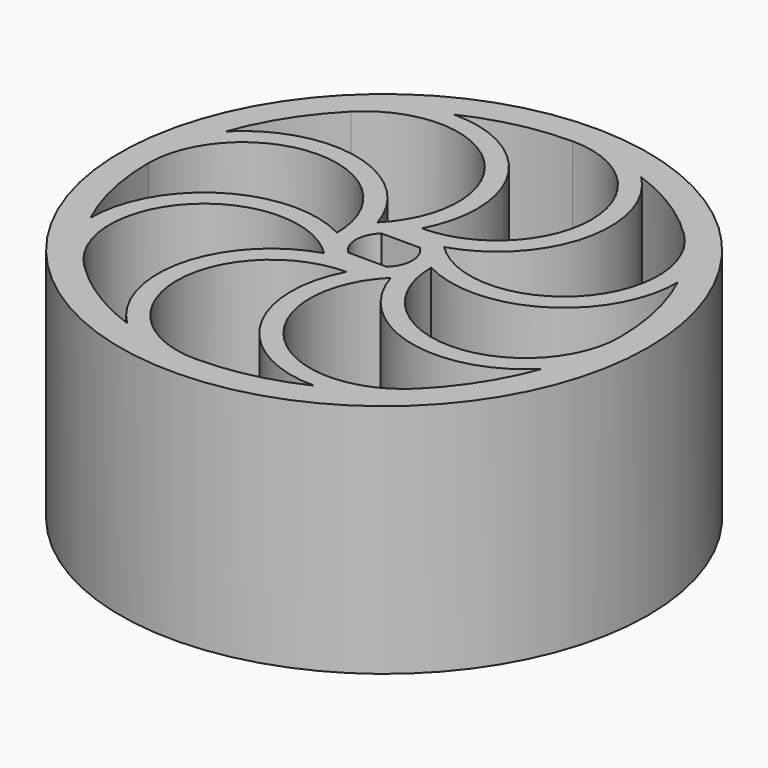
from build123d import *

# Parameters (mm, degrees)
F0_R     = 28
F1_DEPTH = 25
F2_W     = 4.0792156109
F2_H     = 4.4
F3_DEPTH = 30
F4_R     = 5
F4_R_2   = 3.5
F5_DEPTH = 1


# Not quite as in the source:
# - ends of sketch curves that miss each other by under 0.0002 mm in the source are joined


with BuildPart() as f1:
    # F0 (on Top) → F1 (new body)
    with BuildSketch(Plane.XY):
        Circle(F0_R)
        with BuildLine():
            ThreePointArc((22.6064085074, 10.6747503202), (24.3942638, 5.4699080119), (25, 0))
            ThreePointArc((25, 0), (24.6306042082, -4.2817445441), (23.5333330927, -8.4369564149))
            ThreePointArc((23.5333330927, -8.4369564149), (21.1171584026, -13.3815403074), (17.6776695297, -17.6776695297))
            ThreePointArc((17.6776695297, -17.6776695297), (14.3888166579, -20.4441178628), (10.6747503202, -22.6064085074))
            ThreePointArc((10.6747503202, -22.6064085074), (5.4699080119, -24.3942638), (0, -25))
            ThreePointArc((0, -25), (-4.2817445441, -24.6306042082), (-8.4369564149, -23.5333330927))
            ThreePointArc((-8.4369564149, -23.5333330927), (-13.3815403074, -21.1171584026), (-17.6776695297, -17.6776695297))
            ThreePointArc((-17.6776695297, -17.6776695297), (-20.4441178628, -14.3888166579), (-22.6064085074, -10.6747503202))
            ThreePointArc((-22.6064085074, -10.6747503202), (-24.3942638, -5.4699080119), (-25, 0))
            ThreePointArc((-25, 0), (-24.6306042082, 4.2817445441), (-23.5333330927, 8.4369564149))
            ThreePointArc((-23.5333330927, 8.4369564149), (-21.1171584026, 13.3815403074), (-17.6776695297, 17.6776695297))
            ThreePointArc((-17.6776695297, 17.6776695297), (-14.3888166579, 20.4441178628), (-10.6747503202, 22.6064085074))
            ThreePointArc((-10.6747503202, 22.6064085074), (-5.4699080119, 24.3942638), (0, 25))
            ThreePointArc((0, 25), (4.2817445441, 24.6306042082), (8.4369564149, 23.5333330927))
            ThreePointArc((8.4369564149, 23.5333330927), (13.3815403074, 21.1171584026), (17.6776695297, 17.6776695297))
            ThreePointArc((17.6776695297, 17.6776695297), (20.4441178628, 14.3888166579), (22.6064085074, 10.6747503202))
        make_face(mode=Mode.SUBTRACT)
        with BuildLine():
            ThreePointArc((23.5333330927, -8.4369564149), (24.6306042082, -4.2817445441), (25, 0))
            ThreePointArc((25, 0), (15.0015557257, -9.999999879), (5.0000004841, -0.0031114513))
            ThreePointArc((5.0000004841, -0.0031114513), (16.8293380679, 0.3461163718), (22.6064085074, 10.6747503202))
            ThreePointArc((22.6064085074, 10.6747503202), (20.4441178628, 14.3888166579), (17.6776695297, 17.6776695297))
            ThreePointArc((17.6776695297, 17.6776695297), (17.6787695083, 3.5366340557), (3.5377343766, 3.5333341199))
            ThreePointArc((3.5377343766, 3.5333341199), (11.6553978371, 12.1448803043), (8.4369564149, 23.5333330927))
            ThreePointArc((8.4369564149, 23.5333330927), (4.2817445441, 24.6306042082), (0, 25))
            ThreePointArc((0, 25), (9.999999879, 15.0015557257), (0.0031114513, 5.0000004841))
            ThreePointArc((0.0031114513, 5.0000004841), (-0.3461163718, 16.8293380679), (-10.6747503202, 22.6064085074))
            ThreePointArc((-10.6747503202, 22.6064085074), (-14.3888166579, 20.4441178628), (-17.6776695297, 17.6776695297))
            ThreePointArc((-17.6776695297, 17.6776695297), (-3.5366340557, 17.6787695083), (-3.5333341199, 3.5377343766))
            ThreePointArc((-3.5333341199, 3.5377343766), (-12.1448803043, 11.6553978371), (-23.5333330927, 8.4369564149))
            ThreePointArc((-23.5333330927, 8.4369564149), (-24.6306042082, 4.2817445441), (-25, 0))
            ThreePointArc((-25, 0), (-15.0015556407, 9.999999879), (-5.000000484, 0.0031112813))
            ThreePointArc((-5.000000484, 0.0031112813), (-16.8293380679, -0.3461163718), (-22.6064085074, -10.6747503202))
            ThreePointArc((-22.6064085074, -10.6747503202), (-20.4441178628, -14.3888166579), (-17.6776695297, -17.6776695297))
            ThreePointArc((-17.6776695297, -17.6776695297), (-17.6787695083, -3.5366340557), (-3.5377343766, -3.5333341199))
            ThreePointArc((-3.5377343766, -3.5333341199), (-11.6553978371, -12.1448803043), (-8.4369564149, -23.5333330927))
            ThreePointArc((-8.4369564149, -23.5333330927), (-4.2817445441, -24.6306042082), (0, -25))
            ThreePointArc((0, -25), (-9.999999879, -15.0015557257), (-0.0031114513, -5.0000004841))
            ThreePointArc((-0.0031114513, -5.0000004841), (0.3461163718, -16.8293380679), (10.6747503202, -22.6064085074))
            ThreePointArc((10.6747503202, -22.6064085074), (14.3888166579, -20.4441178628), (17.6776695297, -17.6776695297))
            ThreePointArc((17.6776695297, -17.6776695297), (3.5366340557, -17.6787695083), (3.5333341199, -3.5377343766))
            ThreePointArc((3.5333341199, -3.5377343766), (12.1448803043, -11.6553978371), (23.5333330927, -8.4369564149))
        make_face()
    extrude(amount=F1_DEPTH)

    # F2 (on Top) → F3 (cut)
    with BuildSketch(Plane.XY):
        with BuildLine():
            Line((-2.0396078054, -2.2), (-2.0396078054, 2.2))
            ThreePointArc((-2.0396078054, 2.2), (-3, 0), (-2.0396078054, -2.2))
        make_face()
        Rectangle(F2_W, F2_H)
        with BuildLine():
            ThreePointArc((2.0396078054, -2.2), (2.7494384351, -1.2002450966), (3, 0))
            ThreePointArc((3, 0), (2.7494384351, 1.2002450966), (2.0396078054, 2.2))
            Line((2.0396078054, 2.2), (2.0396078054, -2.2))
        make_face()
    extrude(amount=F3_DEPTH, mode=Mode.SUBTRACT)

    # F4 (on Top) → F5 (join)
    with BuildSketch(Plane.XY):
        Circle(F4_R)
        Circle(F4_R_2, mode=Mode.SUBTRACT)
    extrude(amount=-F5_DEPTH)


solid = f1.part
